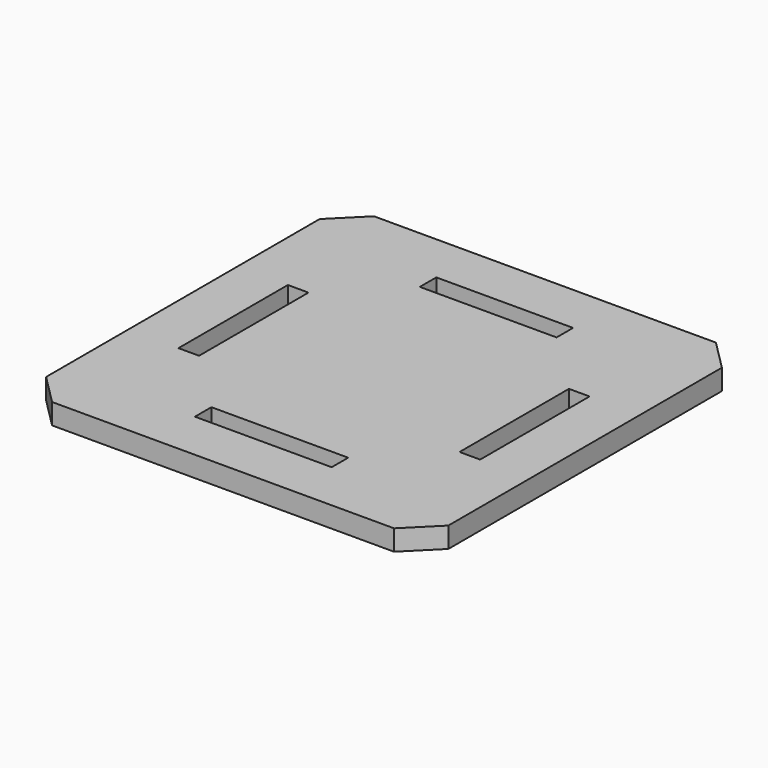
from build123d import *

# Parameters (mm, degrees)
F0_W            = 101.6
F0_H            = 101.6
F1_DEPTH        = 5.207
F2_SIZE         = 7.62
F3_W            = 17.272
F3_H            = 5.207
F3_W_2          = 5.207
F3_H_2          = 17.272
F4_DEPTH        = 25.4
F4_COPIES_COUNT = 4


# Not quite as in the source:
# - a pattern or mirror of a feature is missing from the dataset's text; its kind, count and spacing are read off the source's solid


with BuildPart() as f1:
    # F0 (on Top) → F1 (new body)
    with BuildSketch(Plane.XY):
        Rectangle(F0_W, F0_H)
    extrude(amount=F1_DEPTH)

    # F2
    f2_edges = [f1.edges().sort_by_distance(p)[0] for p in [
        (50.8, -50.8, 2.6035),
        (-50.8, -50.8, 2.6035),
        (50.8, 50.8, 2.6035),
        (-50.8, 50.8, 2.6035),
    ]]
    chamfer(f2_edges, length=F2_SIZE)

    # F3 (on face) → F4 (cut)
    with BuildSketch(Plane.XY.offset(5.207)):
        with Locations((8.636, -35.4965)):
            Rectangle(F3_W, F3_H)
        with Locations((35.4965, -8.636)):
            Rectangle(F3_W_2, F3_H_2)
    f4 = extrude(amount=-F4_DEPTH, mode=Mode.SUBTRACT)

    # F4_copies: F4 ×4 about axis
    f4_copies_axis = Axis((0, 0, 0), (0, 0, 1))
    for i in range(1, F4_COPIES_COUNT):
        add(f4.rotate(f4_copies_axis, i * 360 / F4_COPIES_COUNT), mode=Mode.SUBTRACT)


solid = f1.part
